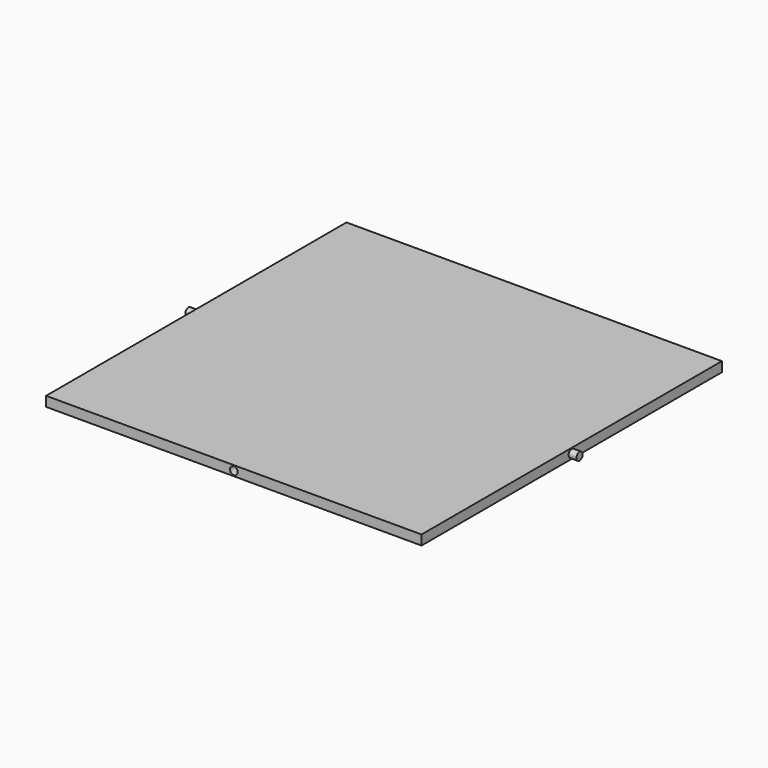
from build123d import *

# Parameters (mm, degrees)
F0_W     = 609.6
F0_H     = 609.6
F1_DEPTH = 7.9375
F2_R     = 6.35
F3_DEPTH = 12.7
F4_R     = 6.35
F5_DEPTH = 12.7
F6_R     = 6.35
F7_DEPTH = 12.7
F8_R     = 6.35
F9_DEPTH = 12.7


# Not quite as in the source:
# - a length typed as a fraction of an inch, garbled in the dataset ("3 / 203.2 mm" for 3/8 in), is restored


with BuildPart() as f1:
    # F0 (on Top) → F1 (new body, symmetric)
    with BuildSketch(Plane.XY):
        Rectangle(F0_W, F0_H)
    extrude(amount=F1_DEPTH, both=True)

    # F2 (on face) → F3 (join)
    with BuildSketch(Plane.YZ.offset(304.8)):
        Circle(F2_R)
    extrude(amount=F3_DEPTH)

    # F4 (on face) → F5 (cut)
    with BuildSketch(Plane.XZ.offset(304.8)):
        Circle(F4_R)
    extrude(amount=-F5_DEPTH, mode=Mode.SUBTRACT)

    # F6 (on face) → F7 (join)
    with BuildSketch(Plane(origin=(-304.8, 0, 0), x_dir=(0, -1, 0), z_dir=(-1, 0, 0))):
        Circle(F6_R)
    extrude(amount=F7_DEPTH)

    # F8 (on face) → F9 (cut)
    with BuildSketch(Plane(origin=(0, 304.8, 0), x_dir=(-1, 0, 0), z_dir=(0, 1, 0))):
        Circle(F8_R)
    extrude(amount=-F9_DEPTH, mode=Mode.SUBTRACT)


solid = f1.part
